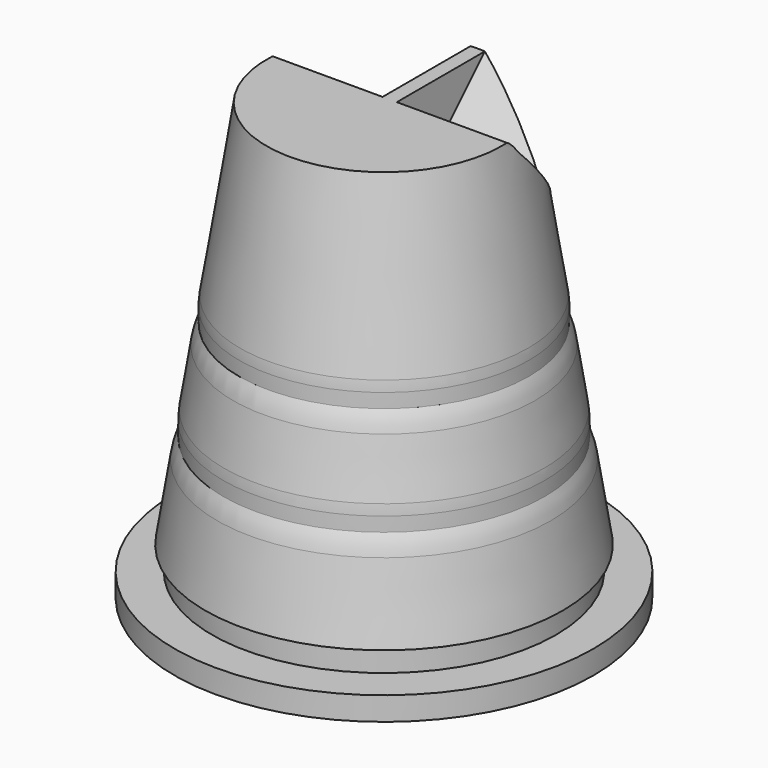
from build123d import *

# Parameters (mm, degrees)
F2_R      = 15.875
F3_DEPTH  = 1.778
F4_W      = 0.889
F4_H      = 1.778
F6_R      = 5.08
F12_DEPTH = 25.4


# Not quite as in the source:
# - a fillet or chamfer that OpenCascade refuses, or shapes differently, is made with other operations: its cross-section is extruded or revolved along the edge and cut away or added


with BuildPart() as f1:
    # F0 (on Front) → F1 (revolve)
    with BuildSketch(Plane.XZ):
        Polygon((8.89, 16.51), (0, 16.51), (0, 3.302), (10.9728, 3.302), align=None)
        Polygon((10.9728, 3.302), (0, 3.302), (0, 1.27), (11.2932307692, 1.27), (10.9728, 1.8250023726), align=None)
        Polygon((11.2932307692, 1.27), (0, 1.27), (0, -4.318), (12.1744153846, -4.318), align=None)
        Polygon((12.1744153846, -4.318), (0, -4.318), (0, -6.35), (12.4948461538, -6.35), (12.1744153846, -5.7949976274), align=None)
        Polygon((12.4948461538, -6.35), (0, -6.35), (0, -16.51), (14.097, -16.51), align=None)
    revolve(axis=Axis((0, 0, 0), (0, 0, -1)))

    # F2 (on face) → F3 (join)
    with BuildSketch(Plane(origin=(0, 0, -16.51), x_dir=(1, 0, 0), z_dir=(0, 0, -1))):
        Circle(F2_R)
    extrude(amount=-F3_DEPTH)

    # F4 (on Front) → F5 (revolve, cut)
    with BuildSketch(Plane.XZ):
        with Locations((13.4747296192, -13.843)):
            Rectangle(F4_W, F4_H)
    revolve(axis=Axis((0, 0, -8.2004386932), (0, 0, -1)), mode=Mode.SUBTRACT)

    # F6
    f6_edges = [f1.edges().sort_by_distance(p)[0] for p in [
        (-12.174415, 0, -4.318),
        (-10.9728, 0, 3.302),
    ]]
    fillet(f6_edges, radius=F6_R)

    # F7: fillet of radius 5.08 on 2 edges, made by hand

    # F7_s1 → F7_t2 (revolve, cut)
    with BuildSketch(Plane.XZ):
        with BuildLine():
            ThreePointArc((10.9728, 1.8250023726), (11.259283136, 1.1139138917), (11.4354988153, 0.367812391))
            Line((11.4354988153, 0.367812391), (11.2932307692, 1.27))
            Line((11.2932307692, 1.27), (10.9728, 1.8250023726))
        make_face()
    revolve(axis=Axis((0, 0, 1.27), (0, 0, -1)), mode=Mode.SUBTRACT)

    # F7_s3 → F7_t4 (revolve, cut)
    with BuildSketch(Plane.XZ):
        with BuildLine():
            ThreePointArc((12.1744153846, -5.7949976274), (12.4608985206, -6.5060861083), (12.6371141999, -7.252187609))
            Line((12.6371141999, -7.252187609), (12.4948461538, -6.35))
            Line((12.4948461538, -6.35), (12.1744153846, -5.7949976274))
        make_face()
    revolve(axis=Axis((0, 0, -6.35), (0, 0, -1)), mode=Mode.SUBTRACT)

    # F11 (on line) → F12 (cut)
    with BuildSketch(Plane(origin=(0, 8.524875, 8.524875), x_dir=(-1, 0, 0), z_dir=(0, 0.7071067812, 0.7071067812))):
        with BuildLine():
            Line((8.8735996043, 11.2926720722), (0.53975, 11.2926720722))
            Line((0.53975, 11.2926720722), (0.53975, 5.3997505037))
            Line((0.53975, 5.3997505037), (7.62, -2.9089047656))
            add(Edge.make_bspline(
                [(8.8735996043, 11.2926720722), (8.9393181622, 8.7279276849), (9.2979393658, 4.1523383564), (7.9516483041, -0.3346072044), (7.62, -2.9089047656)],
                knots=[0, 0, 0, 0, 0.4980817697, 1, 1, 1, 1], degree=3))
        make_face()
        with BuildLine():
            Line((-0.53975, 5.3997505037), (-0.53975, 11.2926720722))
            Line((-0.53975, 11.2926720722), (-8.8735996043, 11.2926720722))
            add(Edge.make_bspline(
                [(-8.8735996043, 11.2926720722), (-8.9393181622, 8.7279276849), (-9.2979393658, 4.1523383564), (-7.9516483041, -0.3346072044), (-7.62, -2.9089047656)],
                knots=[0, 0, 0, 0, 0.4980817697, 1, 1, 1, 1], degree=3))
            Line((-7.62, -2.9089047656), (-0.53975, 5.3997505037))
        make_face()
    extrude(amount=F12_DEPTH, mode=Mode.SUBTRACT)


solid = f1.part
